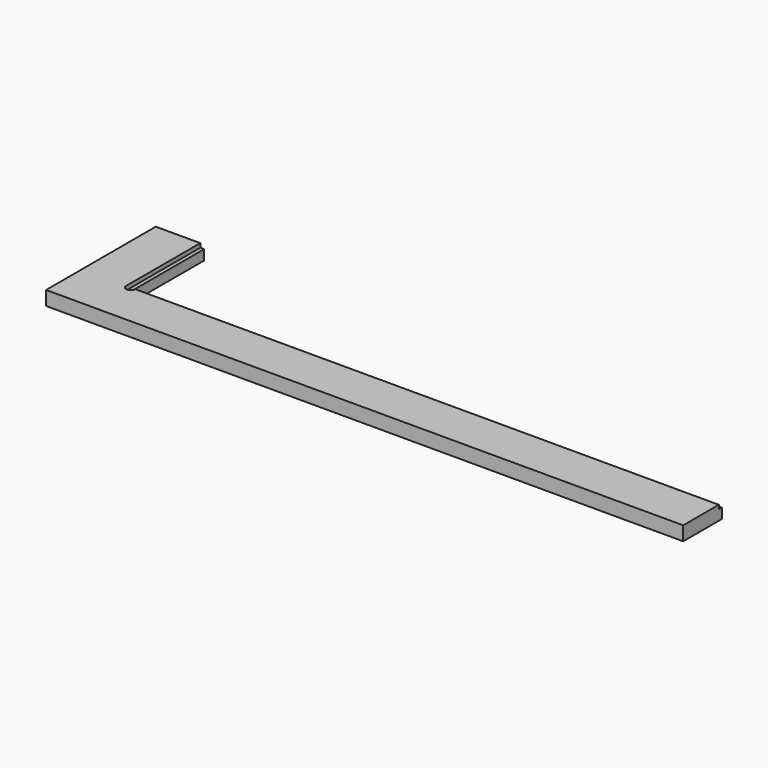
from build123d import *

# Parameters (mm, degrees)
F1_DEPTH = 15.875
F2_DEPTH = 6.35


# Not quite as in the source:
# - a length typed as a fraction of an inch, garbled in the dataset ("3 / 203.2 mm" for 3/8 in), is restored


with BuildPart() as f1:
    # F0 (on Top) → F1 (new body)
    with BuildSketch(Plane.XY):
        with BuildLine():
            Line((927.1, 0), (12.7, 0))
            ThreePointArc((12.7, 0), (11.43, -3.81), (8.128, -6.096))
            Line((8.128, -6.096), (927.1, -6.096))
            Line((927.1, -6.096), (927.1, 0))
        make_face()
        with BuildLine():
            Line((927.1, -6.096), (8.128, -6.096))
            ThreePointArc((8.128, -6.096), (1.016, -13.208), (-6.096, -6.096))
            Line((-6.096, -6.096), (-6.096, 139.7))
            Line((-6.096, 139.7), (-76.2, 139.7))
            Line((-76.2, 139.7), (-76.2, -76.2))
            Line((-76.2, -76.2), (927.1, -76.2))
            Line((927.1, -76.2), (927.1, -6.096))
        make_face()
        with BuildLine():
            ThreePointArc((-6.096, -6.096), (1.016, -13.208), (8.128, -6.096))
            ThreePointArc((8.128, -6.096), (2.54, -5.08), (0, 0))
            Line((0, 0), (0, 139.7))
            Line((0, 139.7), (-6.096, 139.7))
            Line((-6.096, 139.7), (-6.096, -6.096))
        make_face()
    extrude(amount=-F1_DEPTH)

    # F0 (on Top) → F2 (join)
    with BuildSketch(Plane.XY):
        with BuildLine():
            Line((927.1, -6.096), (8.128, -6.096))
            ThreePointArc((8.128, -6.096), (1.016, -13.208), (-6.096, -6.096))
            Line((-6.096, -6.096), (-6.096, 139.7))
            Line((-6.096, 139.7), (-76.2, 139.7))
            Line((-76.2, 139.7), (-76.2, -76.2))
            Line((-76.2, -76.2), (927.1, -76.2))
            Line((927.1, -76.2), (927.1, -6.096))
        make_face()
    extrude(amount=F2_DEPTH)


solid = f1.part
